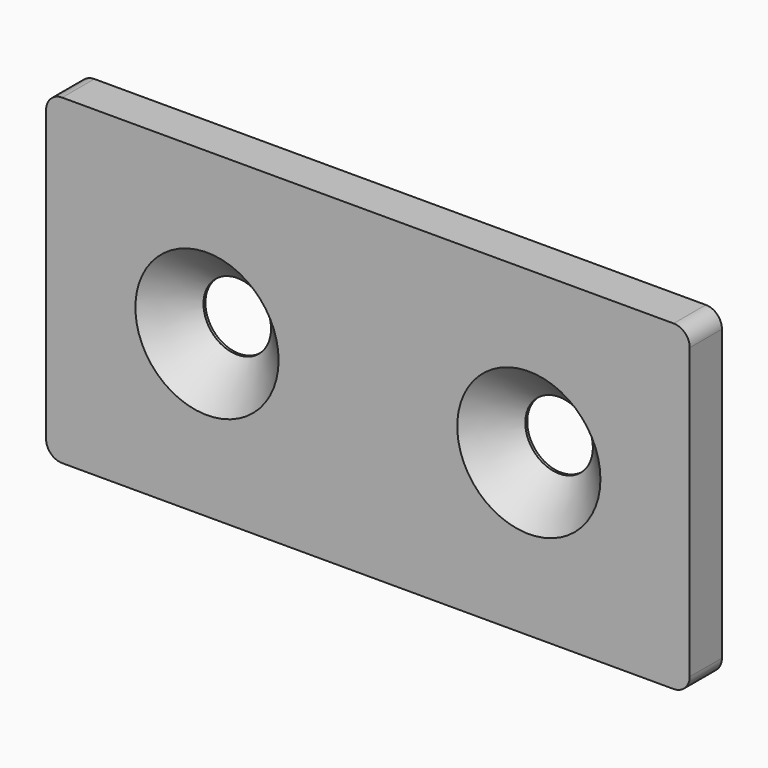
from build123d import *

# Parameters (mm, degrees)
F0_R     = 4.2
F1_DEPTH = 5
F2_SIZE  = 4.7


# Not quite as in the source:
# - a feature names something its author has since deleted; it is built from what else it names


with BuildPart() as f1:
    # F0 (on Front) → F1 (new body)
    with BuildSketch(Plane.XZ):
        with BuildLine():
            Line((58, 20), (-18, 20))
            ThreePointArc((-18, 20), (-19.4142135624, 19.4142135624), (-20, 18))
            Line((-20, 18), (-20, -18))
            ThreePointArc((-20, -18), (-19.4142135624, -19.4142135624), (-18, -20))
            Line((-18, -20), (58, -20))
            ThreePointArc((58, -20), (59.4142135624, -19.4142135624), (60, -18))
            Line((60, -18), (60, 18))
            ThreePointArc((60, 18), (59.4142135624, 19.4142135624), (58, 20))
        make_face()
        Circle(F0_R, mode=Mode.SUBTRACT)
        with Locations((40, 0)):
            Circle(F0_R, mode=Mode.SUBTRACT)
    extrude(amount=F1_DEPTH)

    # F2
    f2_edges = [f1.edges().sort_by_distance(p)[0] for p in [
        (-4.2, -5, 0),
        (35.8, -5, 0),
    ]]
    chamfer(f2_edges, length=F2_SIZE)


solid = f1.part
